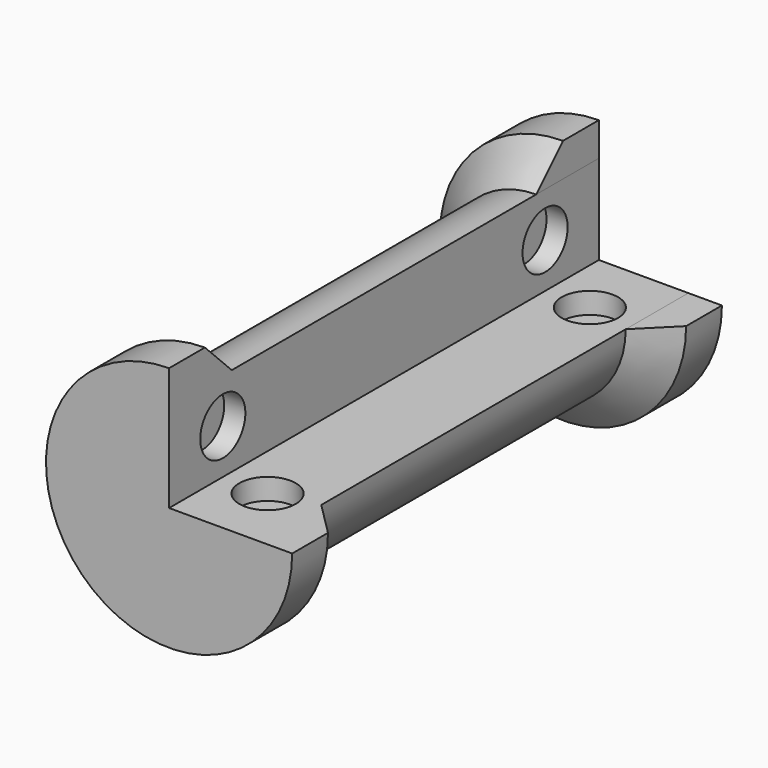
from build123d import *

# Parameters (mm, degrees)
F0_R          = 25.4
F1_DEPTH      = 76.2
F2_R          = 34.925
F2_R_2        = 25.4
F4_DEPTH      = 25.4
F3_R          = 34.925
F3_R_2        = 25.4
F5_DEPTH      = 25.4
F6_2_S5_R     = 25.4
F6_2_T6_DEPTH = 51
F7_W          = 48.0628833175
F7_H          = 48.6316718161
F8_DEPTH      = 88.9
F9_R          = 8
F10_DEPTH     = 6
F11_R         = 8
F12_DEPTH     = 6


# Not quite as in the source:
# - a fillet or chamfer that OpenCascade refuses, or shapes differently, is made with other operations: its cross-section is extruded or revolved along the edge and cut away or added


with BuildPart() as f1:
    # F0 (on Front) → F1 (new body, symmetric)
    with BuildSketch(Plane.XZ):
        Circle(F0_R)
    extrude(amount=F1_DEPTH, both=True)

    # F2 (on face) → F4 (join)
    with BuildSketch(Plane.XZ.offset(76.2)):
        Circle(F2_R)
        Circle(F2_R_2, mode=Mode.SUBTRACT)
    extrude(amount=-F4_DEPTH)

    # F6#2: chamfer of 12.7 on 1 edges, made by hand


with BuildPart() as f5:
    # F3 (on face) → F5 (new body)
    with BuildSketch(Plane(origin=(0, 76.2, 0), x_dir=(-1, 0, 0), z_dir=(0, 1, 0))):
        Circle(F3_R)
        Circle(F3_R_2, mode=Mode.SUBTRACT)
    extrude(amount=-F5_DEPTH)

    # F6: chamfer of 12.7 on 1 edges, made by hand

    # F6_s1 → F6_t2 (revolve, cut)
    with BuildSketch(Plane.XY):
        Polygon((-34.925, 63.5), (-22.225, 50.8), (-34.925, 50.8), align=None)
    revolve(axis=Axis((0, 50.8, 0), (0, 1, 0)), mode=Mode.SUBTRACT)


with BuildPart() as f6_2_tool2:
    # F6_2_s3 → F6_2_t4 (revolve)
    with BuildSketch(Plane.XY):
        Polygon((22.225, -50.8), (34.925, -63.5), (34.925, -50.8), align=None)
    revolve(axis=Axis((0, -50.8, 0), (0, -1, 0)))

    # F6_2_s5 → F6_2_t6 (cut, symmetric)
    with BuildSketch(Plane.XZ.offset(57.2)):
        Circle(F6_2_S5_R)
    extrude(amount=F6_2_T6_DEPTH, both=True, mode=Mode.SUBTRACT)


with BuildPart() as f1_1:
    add(f1.part)

    # F6_2_t1: cut F6_2_tool2
    add(f6_2_tool2.part, mode=Mode.SUBTRACT)


with BuildPart() as f8_tool:
    # F7 (on Front) → F8 (new body, symmetric)
    with BuildSketch(Plane.XZ):
        with Locations((24.0314416587, 24.3158359081)):
            Rectangle(F7_W, F7_H)
    extrude(amount=F8_DEPTH, both=True)


with BuildPart() as f1_2:
    add(f1_1.part)

    # F8: cut by f8_tool
    add(f8_tool.part, mode=Mode.SUBTRACT)

    # F9 (on face) → F10 (cut)
    with BuildSketch(Plane.YZ):
        with Locations((-57.15, 12.7)):
            Circle(F9_R)
        with Locations((57.15, 12.7)):
            Circle(F9_R)
    extrude(amount=-F10_DEPTH, mode=Mode.SUBTRACT)

    # F11 (on face) → F12 (cut)
    with BuildSketch(Plane.XY):
        with Locations((12.7, -57.15)):
            Circle(F11_R)
        with Locations((12.7, 57.15)):
            Circle(F11_R)
    extrude(amount=-F12_DEPTH, mode=Mode.SUBTRACT)


with BuildPart() as f5_1:
    add(f5.part)

    # F8: cut by f8_tool
    add(f8_tool.part, mode=Mode.SUBTRACT)


solid = Compound([f1_2.part, f5_1.part])
